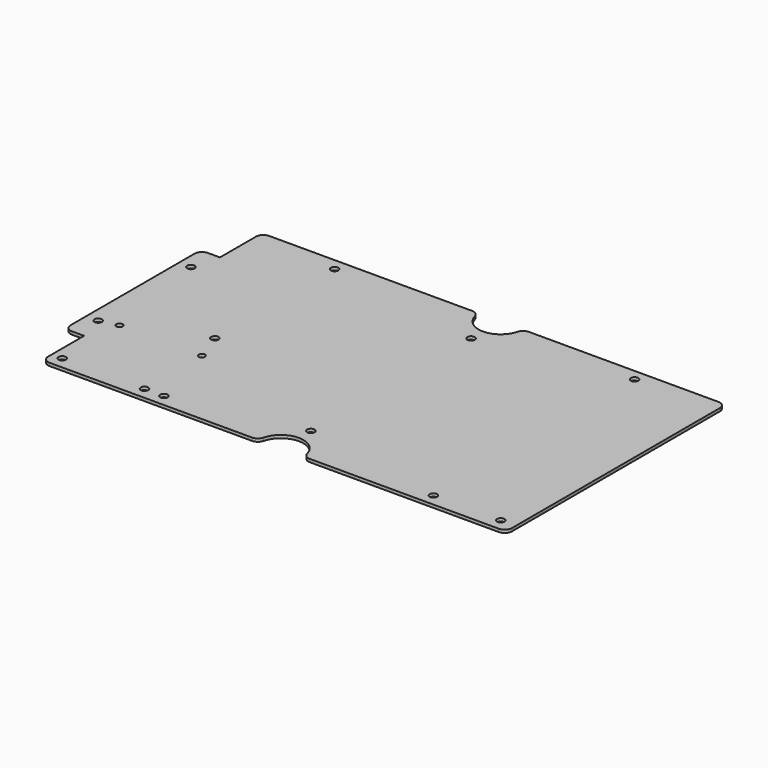
from build123d import *

# Parameters (mm, degrees)
F1_DEPTH = 2
F2_D     = 5
F2_DEPTH = 22.4
F2_TIP   = 1.5021515476
F3_D     = 4.2
F3_DEPTH = 22.4
F3_TIP   = 1.2618073
F4_D     = 5
F4_DEPTH = 22.4
F4_TIP   = 1.5021515476
F5_D     = 5
F5_DEPTH = 22.4
F5_TIP   = 1.5021515476


# Not quite as in the source:
# - a feature names something its author has since deleted; it is built from what else it names


with BuildPart() as f1:
    # F0 (on Top) → F1 (new body)
    with BuildSketch(Plane.XY):
        with BuildLine():
            Line((-19.0027786864, 90.978695631), (-154.5, 90.978695631))
            ThreePointArc((-154.5, 90.978695631), (-158.0355339059, 89.514229537), (-159.5, 85.978695631))
            Line((-159.5, 85.978695631), (-159.5, 55.978695631))
            Line((-159.5, 55.978695631), (-167.5, 55.978695631))
            ThreePointArc((-167.5, 55.978695631), (-171.0355339059, 54.514229537), (-172.5, 50.978695631))
            Line((-172.5, 50.978695631), (-172.5, -52.5))
            ThreePointArc((-172.5, -52.5), (-171.0355339059, -56.0355339059), (-167.5, -57.5))
            Line((-167.5, -57.5), (-159.5, -57.5))
            Line((-159.5, -57.5), (-159.5, -87.5))
            ThreePointArc((-159.5, -87.5), (-158.0355339059, -91.0355339059), (-154.5, -92.5))
            Line((-154.5, -92.5), (-19.364916731, -92.5))
            ThreePointArc((-19.364916731, -92.5), (-16.3030545526, -91.4528470752), (-14.5236875483, -88.75))
            ThreePointArc((-14.5236875483, -88.75), (0, -77.5), (14.5236875483, -88.75))
            ThreePointArc((14.5236875483, -88.75), (16.3030545526, -91.4528470752), (19.364916731, -92.5))
            Line((19.364916731, -92.5), (145.5, -92.5))
            ThreePointArc((145.5, -92.5), (149.0355339059, -91.0355339059), (150.5, -87.5))
            Line((150.5, -87.5), (150.5, 85.978695631))
            ThreePointArc((150.5, 85.978695631), (149.0355339059, 89.514229537), (145.5, 90.978695631))
            Line((145.5, 90.978695631), (19.0027786864, 90.978695631))
            ThreePointArc((19.0027786864, 90.978695631), (15.9500309398, 89.9385859319), (14.1673602092, 87.2509881092))
            ThreePointArc((14.1673602092, 87.2509881092), (0, 76.329125717), (-14.1673602092, 87.2509881092))
            ThreePointArc((-14.1673602092, 87.2509881092), (-15.9500309398, 89.9385859319), (-19.0027786864, 90.978695631))
        make_face()
    extrude(amount=F1_DEPTH)

    # F2
    with Locations(Plane(origin=(0, 0, 0), x_dir=(1, 0, 0), z_dir=(0, 0, -1))):
        with Locations((-104.5, -82.978695631), (95.5, -83.5), (162.5, -84.5), (140.5, 84.5), (95.5, 84.5), (-97.5, 84.5632106066), (-152.5, 84.5)):
            Hole(F2_D / 2, depth=F2_DEPTH)
            with Locations((0, 0, -(F2_DEPTH + F2_TIP / 2))):  # 118° drill point
                Cone(0, F2_D / 2, F2_TIP, mode=Mode.SUBTRACT)

    # F3
    with Locations(Plane(origin=(0, 0, 0), x_dir=(1, 0, 0), z_dir=(0, 0, -1))):
        with Locations((-97.5, 36.6775505245), (-152.5, 36.6775505245)):
            Hole(F3_D / 2, depth=F3_DEPTH)
            with Locations((0, 0, -(F3_DEPTH + F3_TIP / 2))):  # 118° drill point
                Cone(0, F3_D / 2, F3_TIP, mode=Mode.SUBTRACT)

    # F4
    with Locations(Plane(origin=(0, 0, 0), x_dir=(1, 0, 0), z_dir=(0, 0, -1))):
        with Locations((-164.5, -37.978695631), (-164.5, 39.5), (-104.5, 17.021304369), (0, 67.5), (0, -66.329125717), (95.5, -83.5), (95.5, 84.5), (140.5, 84.5), (162.5, -84.5)):
            Hole(F4_D / 2, depth=F4_DEPTH)
            with Locations((0, 0, -(F4_DEPTH + F4_TIP / 2))):  # 118° drill point
                Cone(0, F4_D / 2, F4_TIP, mode=Mode.SUBTRACT)

    # F5
    with Locations(Plane(origin=(0, 0, 0), x_dir=(1, 0, 0), z_dir=(0, 0, -1))):
        with Locations((-84.5, 84.5632106066)):
            Hole(F5_D / 2, depth=F5_DEPTH)
            with Locations((0, 0, -(F5_DEPTH + F5_TIP / 2))):  # 118° drill point
                Cone(0, F5_D / 2, F5_TIP, mode=Mode.SUBTRACT)


solid = f1.part
